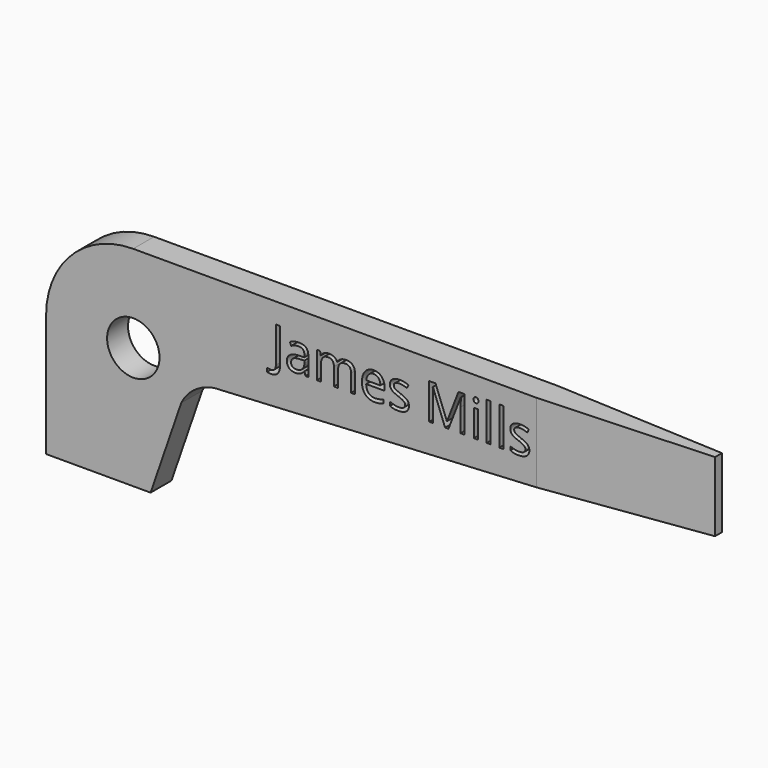
from build123d import *

# Parameters (mm, degrees)
F1_DEPTH     = 2.38125
F2_R         = 2.3876
F3_DEPTH     = 2.38225
F5_DEPTH     = 19.051
F6_TEXT_SIZE = 4.5746176814
F7_DEPTH     = 1.27


# Not quite as in the source:
# - Text() gives the source's letters only with a copy of the font that has no kerning and outlines rounded to 1/6400 em; it was checked with that copy


with BuildPart() as f1:
    # F0 (on Front) → F1 (new body)
    with BuildSketch(Plane.XZ):
        with BuildLine():
            Line((36.2685264707, 24.0700727777), (-16.1189735293, 24.0700727777))
            ThreePointArc((-16.1189735293, 24.0700727777), (-21.731633605, 21.7452328534), (-24.0564735293, 16.1325727777))
            Line((-24.0564735293, 16.1325727777), (-24.0564735293, 5.0200727777))
            Line((-24.0564735293, 5.0200727777), (-14.5314735293, 5.0200727777))
            Line((-14.5314735293, 5.0200727777), (-11.73750988, 13.1323389425))
            ThreePointArc((-11.73750988, 13.1323389425), (-10.2452699326, 14.7600168729), (-8.1141293049, 15.3382513672))
            Line((-8.1141293049, 15.3382513672), (36.2685264707, 17.7200727777))
            Line((36.2685264707, 17.7200727777), (36.2685264707, 24.0700727777))
        make_face()
    extrude(amount=F1_DEPTH)

    # F2 (on face) → F3 (cut, through all)
    with BuildSketch(Plane.XZ.offset(2.38125)):
        with Locations((-16.1062836731, 16.1198727777)):
            Circle(F2_R)
    extrude(amount=-F3_DEPTH, mode=Mode.SUBTRACT)

    # F4 (on face) → F5 (cut, through all)
    with BuildSketch(Plane.XY.offset(24.0700727777)):
        Polygon((36.2685264707, 0), (20.6422731162, 0), (36.2685264707, -0.79375), align=None)
        Polygon((36.2685264707, -2.38125), (36.2685264707, -1.5875), (20.6422731162, -2.38125), align=None)
    extrude(amount=-F5_DEPTH, mode=Mode.SUBTRACT)

    # F6 (on face) → F7 (cut)
    with BuildSketch(Plane.XZ.offset(2.38125)):
        with Locations((-3.5438735222, 18.9693365246)):
            Text('James Mills', F6_TEXT_SIZE, font='Open Sans', text_align=(TextAlign.LEFT, TextAlign.BOTTOM))
    extrude(amount=-F7_DEPTH, mode=Mode.SUBTRACT)


solid = f1.part
